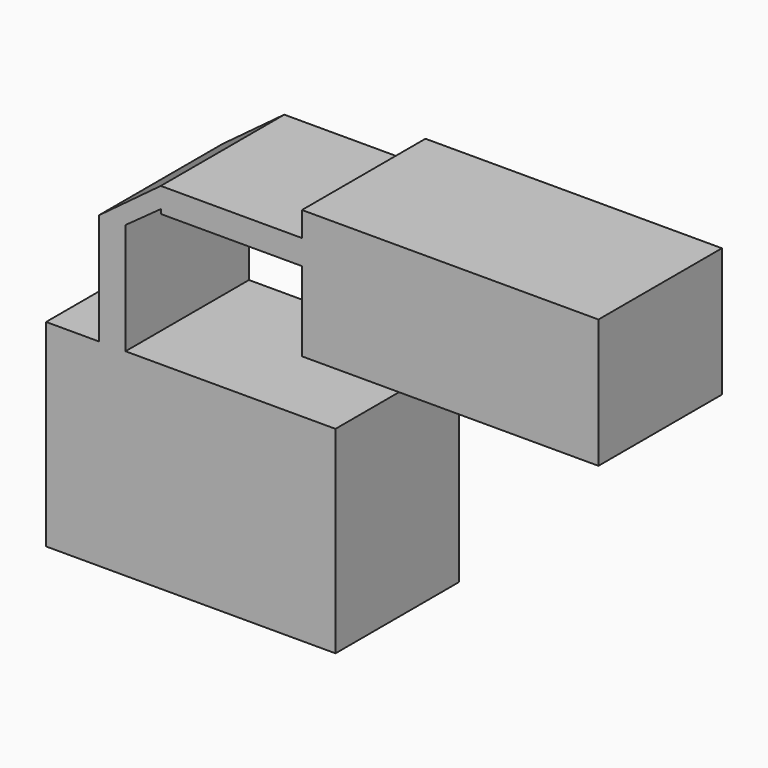
from build123d import *

# Parameters (mm, degrees)
F0_W     = 4.3562594801
F0_H     = 11.6166975349
F0_H_2   = 6.6796019673
F0_W_2   = 8.1316875294
F0_H_3   = 4.0658414364
F0_H_4   = 2.6137568057
F1_DEPTH = 25.4


with BuildPart() as f1:
    # F0 (on Front) → F1 (new body)
    with BuildSketch(Plane.XZ):
        with Locations((-31.219872646, 17.5702543929)):
            Rectangle(F0_W, F0_H)
        Polygon((-33.3980023861, 11.7619056255), (-42.1105250716, 11.7619056255), (-42.1105250716, -20.7648463547), (5.517931655, -20.7648463547), (5.517931655, 11.7619056255), (-29.041742906, 11.7619056255), (-29.041742906, 9.1481488198), (-33.3980023861, 9.1481488198), align=None)
        Polygon((0, 41.6749008), (0, 37.6090556383), (8.1316875294, 37.6090556383), (8.1316875294, 33.5432142019), (0, 33.5432142019), (0, 20.474428311), (48.790127039, 20.474428311), (48.790127039, 41.6749008), align=None)
        Polygon((-18.5867156833, 37.6090556383), (-23.2333932072, 34.2531229749), (-23.2333932072, 33.5432142019), (0, 33.5432142019), (0, 37.6090556383), align=None)
        with Locations((-31.219872646, 26.718404144)):
            Rectangle(F0_W, F0_H_2)
        with Locations((4.0658437647, 35.5761349201)):
            Rectangle(F0_W_2, F0_H_3)
        Polygon((-23.2333932072, 37.6090556383), (-33.3980023861, 30.0582051277), (-29.041742906, 30.0582051277), (-23.2333932072, 34.2531229749), align=None)
        with Locations((-31.219872646, 10.4550272226)):
            Rectangle(F0_W, F0_H_4)
        Polygon((-18.5867156833, 37.6090556383), (-23.2333932072, 37.6090556383), (-23.2333932072, 34.2531229749), align=None)
    extrude(amount=F1_DEPTH)


solid = f1.part
